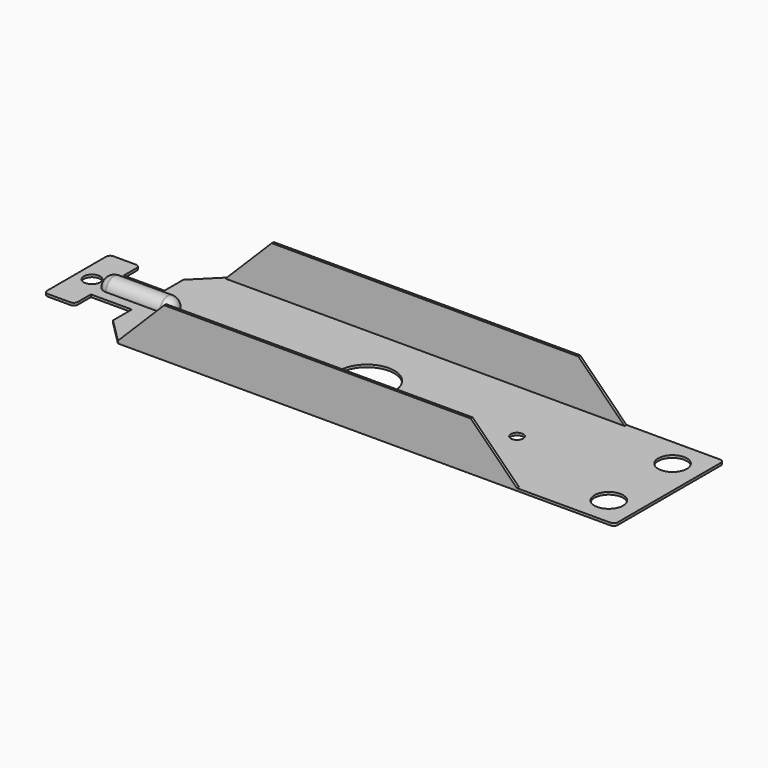
from build123d import *

# Parameters (mm, degrees)
F0_R     = 4.445
F0_R_2   = 8.5725
F0_R_3   = 1.905
F0_W     = 17.4625
F0_H     = 12.7
F0_W_2   = 12.7
F1_DEPTH = 0.762
F3_DEPTH = 0.762
F4_W     = 16.51
F4_H     = 2.921
F5_DEPTH = 25.4
F6_ANGLE = 180


# Not quite as in the source:
# - a pattern or mirror of a feature is missing from the dataset's text; its kind, count and spacing are read off the source's solid


with BuildPart() as f1:
    # F0 (on Top) → F1 (new body)
    with BuildSketch(Plane.XY):
        with BuildLine():
            Line((79.6925, 21.2725), (-73.3425, 21.2725))
            Line((-73.3425, 21.2725), (-80.9625, 13.6525))
            Line((-80.9625, 13.6525), (-80.9625, 6.35))
            Line((-80.9625, 6.35), (-63.5, 6.35))
            Line((-63.5, 6.35), (-63.5, -6.35))
            Line((-63.5, -6.35), (-80.9625, -6.35))
            Line((-80.9625, -6.35), (-80.9625, -13.6525))
            Line((-80.9625, -13.6525), (-73.3425, -21.2725))
            Line((-73.3425, -21.2725), (79.6925, -21.2725))
            ThreePointArc((79.6925, -21.2725), (80.5905256121, -20.9005256121), (80.9625, -20.0025))
            Line((80.9625, -20.0025), (80.9625, 20.0025))
            ThreePointArc((80.9625, 20.0025), (80.5905256121, 20.9005256121), (79.6925, 21.2725))
        make_face()
        with Locations((72.0725, -12.3825)):
            Circle(F0_R, mode=Mode.SUBTRACT)
        with Locations((-13.0175, 0)):
            Circle(F0_R_2, mode=Mode.SUBTRACT)
        with Locations((33.655, 0)):
            Circle(F0_R_3, mode=Mode.SUBTRACT)
        with Locations((72.0725, 12.3825)):
            Circle(F0_R, mode=Mode.SUBTRACT)
        with Locations((-72.23125, 0)):
            Rectangle(F0_W, F0_H)
        with Locations((-87.3125, 0)):
            Rectangle(F0_W_2, F0_H)
        with BuildLine():
            Line((-93.6625, -6.35), (-93.6625, 6.35))
            Line((-93.6625, 6.35), (-98.425, 6.35))
            Line((-98.425, 6.35), (-98.425, 2.54))
            ThreePointArc((-98.425, 2.54), (-96.6289487758, 1.7960512242), (-95.885, 0))
            ThreePointArc((-95.885, 0), (-96.6289487758, -1.7960512242), (-98.425, -2.54))
            Line((-98.425, -2.54), (-98.425, -6.35))
            Line((-98.425, -6.35), (-93.6625, -6.35))
        make_face()
        with BuildLine():
            Line((-98.425, 6.35), (-93.6625, 6.35))
            Line((-93.6625, 6.35), (-93.6625, 11.43))
            ThreePointArc((-93.6625, 11.43), (-94.0344743879, 12.3280256121), (-94.9325, 12.7))
            Line((-94.9325, 12.7), (-101.9175, 12.7))
            ThreePointArc((-101.9175, 12.7), (-102.8155256121, 12.3280256121), (-103.1875, 11.43))
            Line((-103.1875, 11.43), (-103.1875, -11.43))
            ThreePointArc((-103.1875, -11.43), (-102.8155256121, -12.3280256121), (-101.9175, -12.7))
            Line((-101.9175, -12.7), (-94.9325, -12.7))
            ThreePointArc((-94.9325, -12.7), (-94.0344743879, -12.3280256121), (-93.6625, -11.43))
            Line((-93.6625, -11.43), (-93.6625, -6.35))
            Line((-93.6625, -6.35), (-98.425, -6.35))
            Line((-98.425, -6.35), (-98.425, -2.54))
            ThreePointArc((-98.425, -2.54), (-100.965, 0), (-98.425, 2.54))
            Line((-98.425, 2.54), (-98.425, 6.35))
        make_face()
    extrude(amount=F1_DEPTH)

    # F2 (on face) → F3 (join)
    with BuildSketch(Plane.XZ.offset(21.2725)):
        Polygon((-58.9740902063, 15.1304097937), (-73.3425, 0.762), (50.6443195874, 0.762), (36.2759097937, 15.1304097937), align=None)
    f3 = extrude(amount=-F3_DEPTH)

    # F3_copies: F3 across plane
    add(f3.mirror(Plane.ZX))

    # F4 (on face) → F5 (cut)
    with BuildSketch(Plane.XY.offset(0.762)):
        with BuildLine():
            Line((-91.44, 0), (-91.44, 2.921))
            ThreePointArc((-91.44, 2.921), (-93.5054589078, 2.0654589078), (-94.361, 0))
            Line((-94.361, 0), (-91.44, 0))
        make_face()
        with BuildLine():
            Line((-91.44, -2.921), (-91.44, 0))
            Line((-91.44, 0), (-94.361, 0))
            ThreePointArc((-94.361, 0), (-93.5054589078, -2.0654589078), (-91.44, -2.921))
        make_face()
        with Locations((-83.185, 1.4605)):
            Rectangle(F4_W, F4_H)
        with BuildLine():
            Line((-72.009, 0), (-74.93, 0))
            Line((-74.93, 0), (-74.93, -2.921))
            ThreePointArc((-74.93, -2.921), (-72.8645410922, -2.0654589078), (-72.009, 0))
        make_face()
        with BuildLine():
            ThreePointArc((-72.009, 0), (-72.8645410922, 2.0654589078), (-74.93, 2.921))
            Line((-74.93, 2.921), (-74.93, 0))
            Line((-74.93, 0), (-72.009, 0))
        make_face()
        with Locations((-83.185, -1.4605)):
            Rectangle(F4_W, F4_H)
    extrude(amount=-F5_DEPTH, mode=Mode.SUBTRACT)

    # F4 (on face) → F6 (revolve)
    with BuildSketch(Plane.XY.offset(0.762)):
        with BuildLine():
            Line((-71.755, 0), (-72.009, 0))
            ThreePointArc((-72.009, 0), (-72.8645410922, -2.0654589078), (-74.93, -2.921))
            ThreePointArc((-74.93, -2.921), (-74.754023638, -2.9918379952), (-74.6762032813, -3.16484))
            ThreePointArc((-74.6762032813, -3.16484), (-72.5969301787, -2.1534646988), (-71.755, 0))
        make_face()
        with BuildLine():
            ThreePointArc((-74.6762032813, -3.16484), (-74.754023638, -2.9918379952), (-74.93, -2.921))
            Line((-74.93, -2.921), (-74.93, -3.175))
            ThreePointArc((-74.93, -3.175), (-74.803, -3.1724589832), (-74.6762032813, -3.16484))
        make_face()
        with BuildLine():
            Line((-74.93, -3.175), (-74.93, -2.921))
            ThreePointArc((-74.93, -2.921), (-75.1096051224, -2.9953948776), (-75.184, -3.175))
            Line((-75.184, -3.175), (-74.93, -3.175))
        make_face()
        with BuildLine():
            Line((-74.93, -2.921), (-91.44, -2.921))
            ThreePointArc((-91.44, -2.921), (-91.2603948776, -2.9953948776), (-91.186, -3.175))
            Line((-91.186, -3.175), (-75.184, -3.175))
            ThreePointArc((-75.184, -3.175), (-75.1096051224, -2.9953948776), (-74.93, -2.921))
        make_face()
        with BuildLine():
            ThreePointArc((-91.186, -3.175), (-91.2603948776, -2.9953948776), (-91.44, -2.921))
            Line((-91.44, -2.921), (-91.44, -3.175))
            Line((-91.44, -3.175), (-91.186, -3.175))
        make_face()
        with BuildLine():
            Line((-91.44, -3.175), (-91.44, -2.921))
            ThreePointArc((-91.44, -2.921), (-91.615976362, -2.9918379952), (-91.6937967187, -3.16484))
            ThreePointArc((-91.6937967187, -3.16484), (-91.567, -3.1724589832), (-91.44, -3.175))
        make_face()
        with BuildLine():
            ThreePointArc((-91.44, -2.921), (-93.5054589078, -2.0654589078), (-94.361, 0))
            Line((-94.361, 0), (-94.615, 0))
            ThreePointArc((-94.615, 0), (-93.7730698213, -2.1534646988), (-91.6937967187, -3.16484))
            ThreePointArc((-91.6937967187, -3.16484), (-91.615976362, -2.9918379952), (-91.44, -2.921))
        make_face()
    revolve(axis=Axis((-83.185, 0, 0.762), (-1, 0, 0)), revolution_arc=F6_ANGLE)


solid = f1.part
